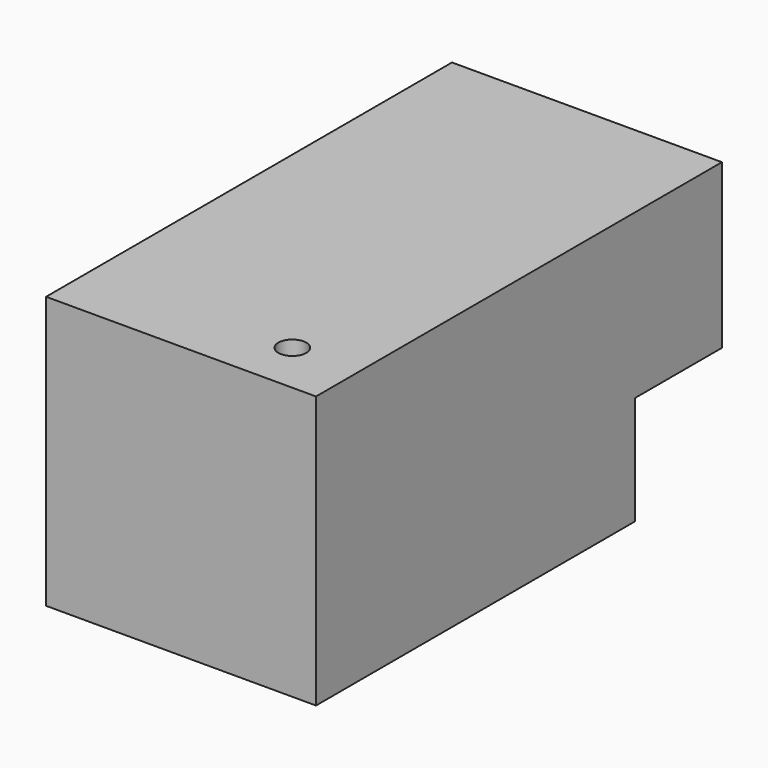
from build123d import *

# Parameters (mm, degrees)
F0_W     = 63.119
F0_H     = 63.627
F1_DEPTH = 118.6434
F2_W     = 25.4
F2_H     = 25.4
F3_DEPTH = 63.119
F4_R     = 3.2639
F5_DEPTH = 63.627
F6_R     = 7.9375
F7_DEPTH = 1.5494


# Not quite as in the source:
# - a feature names something its author has since deleted; it is built from what else it names


with BuildPart() as f1:
    # F0 (on Front) → F1 (new body)
    with BuildSketch(Plane.XZ):
        with Locations((-8.3619841438, 9.8403063603)):
            Rectangle(F0_W, F0_H)
    extrude(amount=F1_DEPTH)

    # F2 (on face) → F3 (cut, through all)
    with BuildSketch(Plane.YZ.offset(23.1975158562)):
        with Locations((-12.7, -9.2731936397)):
            Rectangle(F2_W, F2_H)
    extrude(amount=-F3_DEPTH, mode=Mode.SUBTRACT)

    # F4 (on face) → F5 (cut, through all)
    with BuildSketch(Plane(origin=(0, 0, -21.9731936397), x_dir=(1, 0, 0), z_dir=(0, 0, -1))):
        with Locations((7.7937371098, 106.303319335)):
            Circle(F4_R)
    extrude(amount=-F5_DEPTH, mode=Mode.SUBTRACT)

    # F6 (on face) → F7 (cut)
    with BuildSketch(Plane(origin=(0, 0, -21.9731936397), x_dir=(1, 0, 0), z_dir=(0, 0, -1))):
        with Locations((7.7937371098, 106.303319335)):
            Circle(F6_R)
    extrude(amount=-F7_DEPTH, mode=Mode.SUBTRACT)


solid = f1.part
